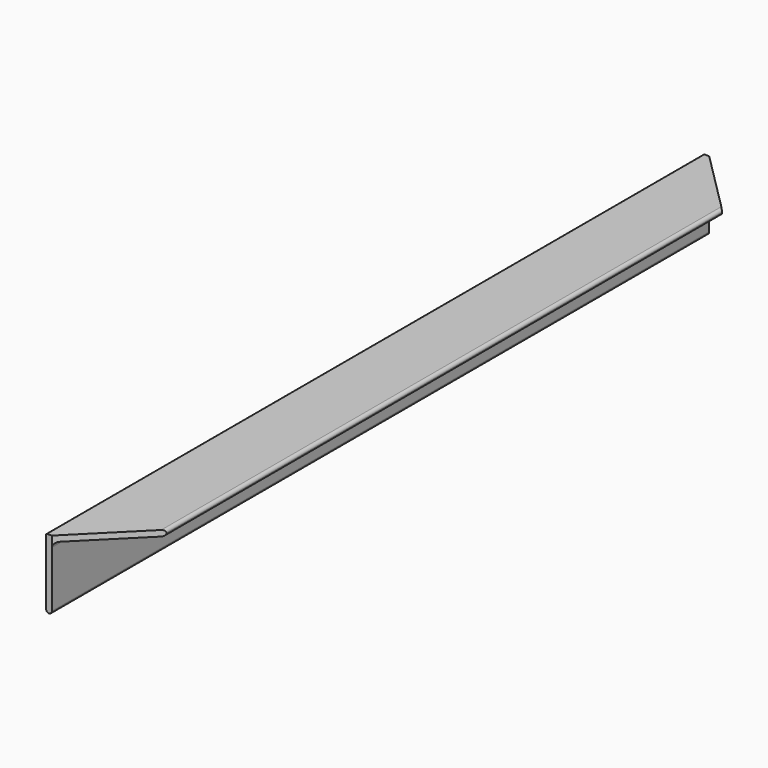
from build123d import *

# Parameters (mm, degrees)
F1_DEPTH = 450.85
F2_R     = 5.08
F4_DEPTH = 76.201
F5_R     = 3.17499
F6_R     = 1.397


# Not quite as in the source:
# - a fillet or chamfer is up to 0.001 mm smaller than in the source, because OpenCascade refuses the exact size


with BuildPart() as f1:
    # F0 (on Front) → F1 (new body, symmetric)
    with BuildSketch(Plane.XZ):
        Polygon((76.2, 0), (0, 0), (0, -76.2), (6.35, -76.2), (6.35, -6.35), (76.2, -6.35), align=None)
    extrude(amount=F1_DEPTH, both=True)

    # F2
    f2_edges = [f1.edges().sort_by_distance(p)[0] for p in [
        (6.35, 0, -6.35),
    ]]
    fillet(f2_edges, radius=F2_R)

    # F3 (on Top) → F4 (cut, through all)
    with BuildSketch(Plane.XY):
        Polygon((76.2, 381), (76.2, 450.85), (6.35, 450.85), align=None)
        Polygon((76.2, -450.85), (76.2, -381), (6.35, -450.85), align=None)
    extrude(amount=-F4_DEPTH, mode=Mode.SUBTRACT)

    # F5 (radius 3.175 in the source; OpenCascade refuses exactly that, so slightly less here)
    f5_edges = [f1.edges().sort_by_distance(p)[0] for p in [
        (76.2, 0, -6.35),
        (76.2, 0, 0),
        (0, 0, -76.2),
        (6.35, 0, -76.2),
    ]]
    fillet(f5_edges, radius=F5_R)

    # F6
    f6_edges = [f1.edges().sort_by_distance(p)[0] for p in [
        (0, 0, 0),
    ]]
    fillet(f6_edges, radius=F6_R)


solid = f1.part
